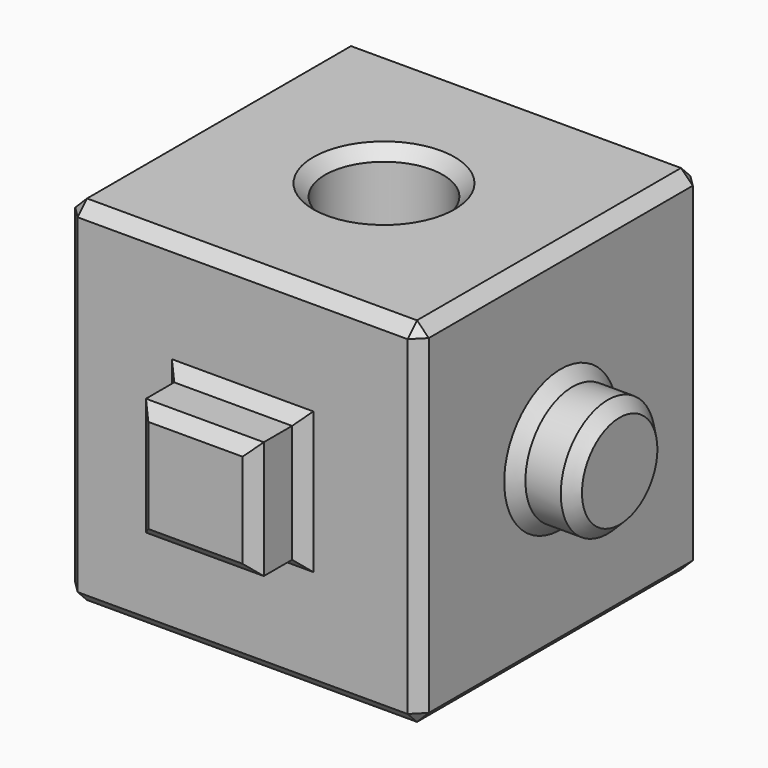
from build123d import *

# Parameters (mm, degrees)
F0_W     = 76.2
F0_H     = 76.2
F1_DEPTH = 76.2
F2_W     = 25.4
F2_H     = 25.4
F3_DEPTH = 12.7
F4_R     = 12.7
F5_DEPTH = 12.7
F7_D     = 25.4
F8_SIZE  = 2.54


with BuildPart() as f1:
    # F0 (on Front) → F1 (new body)
    with BuildSketch(Plane.XZ):
        with Locations((2.74146, 5.687511)):
            Rectangle(F0_W, F0_H)
    extrude(amount=-F1_DEPTH)

    # F2 (on face) → F3 (join)
    with BuildSketch(Plane.XZ):
        with Locations((2.74146, 5.687511)):
            Rectangle(F2_W, F2_H)
    extrude(amount=F3_DEPTH)

    # F4 (on face) → F5 (join)
    with BuildSketch(Plane.YZ.offset(40.84146)):
        with Locations((38.1, 5.687511)):
            Circle(F4_R)
    extrude(amount=F5_DEPTH)

    # F7 (through all)
    with Locations(Plane.XY.offset(43.787511)):
        with Locations((2.74146, 38.1)):
            Hole(F7_D / 2)

    # F8
    f8_edges = [f1.edges().sort_by_distance(p)[0] for p in [
        (40.84146, 38.1, 43.787511),
        (2.74146, 0, 43.787511),
        (2.74146, 76.2, 43.787511),
        (-35.35854, 38.1, 43.787511),
        (-9.95854, 38.1, 43.787511),
        (2.74146, -12.7, 18.387511),
        (-9.95854, -12.7, 5.687511),
        (2.74146, -12.7, -7.012489),
        (15.44146, -12.7, 5.687511),
        (40.84146, 0, 5.687511),
        (2.74146, 0, -32.412489),
        (-35.35854, 0, 5.687511),
        (2.74146, 0, 18.387511),
        (-9.95854, 0, 5.687511),
        (2.74146, 0, -7.012489),
        (15.44146, 0, 5.687511),
        (40.84146, 38.1, -32.412489),
        (40.84146, 76.2, 5.687511),
        (40.84146, 25.4, 5.687511),
        (53.54146, 25.4, 5.687511),
        (-35.35854, 76.2, 5.687511),
        (2.74146, 76.2, -32.412489),
        (-35.35854, 38.1, -32.412489),
        (-9.95854, 38.1, -32.412489),
    ]]
    chamfer(f8_edges, length=F8_SIZE)


solid = f1.part
